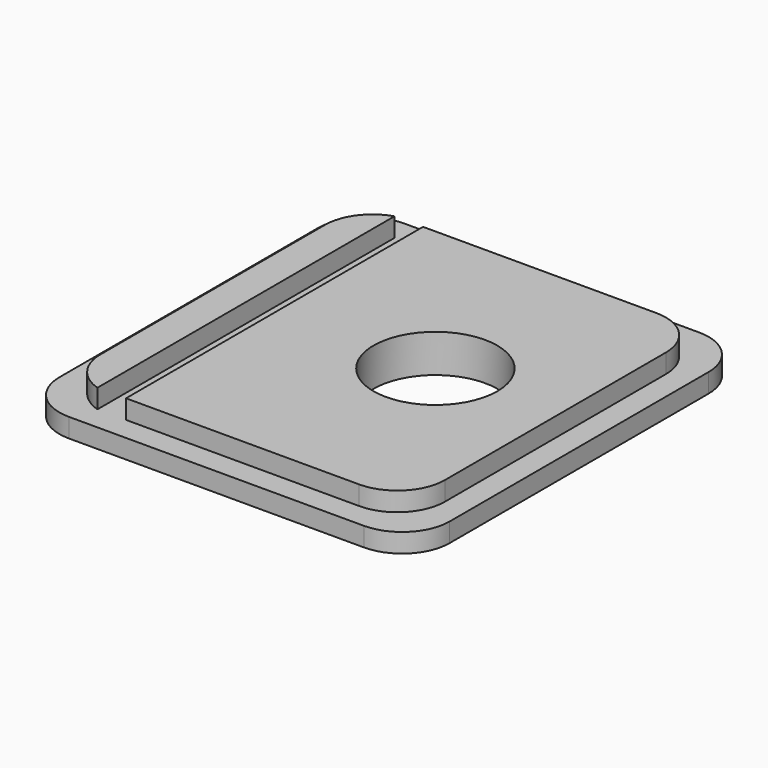
from build123d import *

# Parameters (mm, degrees)
F0_W        = 3
F0_H        = 2.5
F0_H_2      = 39
F1_DEPTH    = 2
F0_W_2      = 3.5
F0_W_3      = 29.5
F0_R        = 6.5
F2_DEPTH    = 4
F3_T1_DEPTH = 13.9242400177
F3_T3_DEPTH = 14.5
F3_T5_DEPTH = 27


# Not quite as in the source:
# - a fillet or chamfer that OpenCascade refuses, or shapes differently, is made with other operations: its cross-section is extruded or revolved along the edge and cut away or added


with BuildPart() as f1:
    # F0 (on Top) → F1 (new body)
    with BuildSketch(Plane.XY):
        Polygon((20.5, -22), (20.5, 22), (-11.5, 22), (-11.5, 19.5), (18, 19.5), (18, -19.5), (-11.5, -19.5), (-11.5, -22), align=None)
        with Locations((-13, 20.75)):
            Rectangle(F0_W, F0_H)
        Polygon((-14.5, 19.5), (-14.5, 22), (-20.5, 22), (-20.5, -22), (-14.5, -22), (-14.5, -19.5), (-18, -19.5), (-18, 19.5), align=None)
        with Locations((-13, -20.75)):
            Rectangle(F0_W, F0_H)
        with Locations((-13, 0)):
            Rectangle(F0_W, F0_H_2)
    extrude(amount=F1_DEPTH)

    # F0 (on Top) → F2 (join)
    with BuildSketch(Plane.XY):
        with Locations((-16.25, 0)):
            Rectangle(F0_W_2, F0_H_2)
        with Locations((3.25, 0)):
            Rectangle(F0_W_3, F0_H_2)
        with Locations((5, 0.5)):
            Circle(F0_R, mode=Mode.SUBTRACT)
    extrude(amount=F2_DEPTH)

    # F3: fillet of radius 5 on 8 edges, made by hand

    # F3_s2 → F3_t1 (cut)
    with BuildSketch(Plane.XY.offset(2)):
        with BuildLine():
            ThreePointArc((-18, 14.7303039929), (-17.0311288741, 17.6883438845), (-14.5, 19.5))
            Line((-14.5, 19.5), (-18, 19.5))
            Line((-18, 19.5), (-18, 14.7303039929))
        make_face()
        with BuildLine():
            ThreePointArc((-18, -14.7303039929), (-17.0311288741, -17.6883438845), (-14.5, -19.5))
            Line((-14.5, -19.5), (-18, -19.5))
            Line((-18, -19.5), (-18, -14.7303039929))
        make_face()
    extrude(amount=F3_T1_DEPTH, mode=Mode.SUBTRACT)

    # F3_s4 → F3_t3 (cut)
    with BuildSketch(Plane.XY.offset(2)):
        with BuildLine():
            ThreePointArc((13, 19.5), (16.5355339059, 18.0355339059), (18, 14.5))
            Line((18, 14.5), (18, 19.5))
            Line((18, 19.5), (13, 19.5))
        make_face()
        with BuildLine():
            ThreePointArc((18, -14.5), (16.5355339059, -18.0355339059), (13, -19.5))
            Line((13, -19.5), (18, -19.5))
            Line((18, -19.5), (18, -14.5))
        make_face()
    extrude(amount=F3_T3_DEPTH, mode=Mode.SUBTRACT)

    # F3_s6 → F3_t5 (cut)
    with BuildSketch(Plane.XY.offset(-12.5)):
        with BuildLine():
            ThreePointArc((-15.5, 22), (-19.0355339059, 20.5355339059), (-20.5, 17))
            Line((-20.5, 17), (-20.5, 22))
            Line((-20.5, 22), (-15.5, 22))
        make_face()
        with BuildLine():
            ThreePointArc((-15.5, -22), (-19.0355339059, -20.5355339059), (-20.5, -17))
            Line((-20.5, -17), (-20.5, -22))
            Line((-20.5, -22), (-15.5, -22))
        make_face()
        with BuildLine():
            ThreePointArc((20.5, 17), (19.0355339059, 20.5355339059), (15.5, 22))
            Line((15.5, 22), (20.5, 22))
            Line((20.5, 22), (20.5, 17))
        make_face()
        with BuildLine():
            ThreePointArc((20.5, -17), (19.0355339059, -20.5355339059), (15.5, -22))
            Line((15.5, -22), (20.5, -22))
            Line((20.5, -22), (20.5, -17))
        make_face()
    extrude(amount=F3_T5_DEPTH, mode=Mode.SUBTRACT)


solid = f1.part
